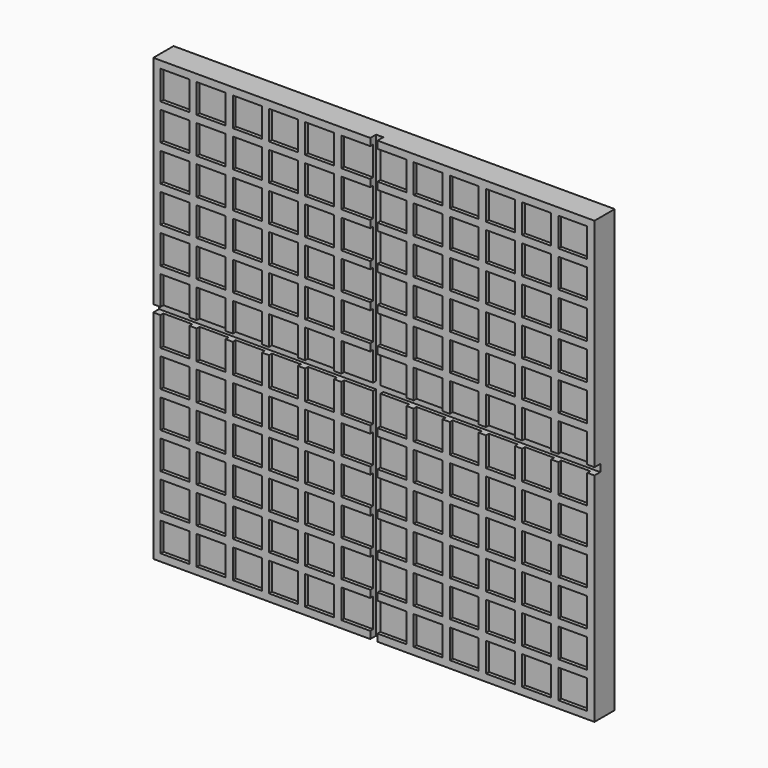
from build123d import *

# Parameters (mm, degrees)
F0_W     = 122
F0_H     = 122
F2_DEPTH = 7
F1_W     = 60
F1_H     = 2
F1_W_2   = 2
F1_H_2   = 60
F3_DEPTH = 7
F4_W     = 8
F4_H     = 8
F5_DEPTH = 1
F6_W     = 60
F6_H     = 2
F6_W_2   = 2
F6_H_2   = 60
F7_DEPTH = 2


# Not quite as in the source:
# - a feature names something its author has since deleted; it is built from what else it names


with BuildPart() as f2:
    # F0 (on Front) → F2 (new body)
    with BuildSketch(Plane.XZ):
        Rectangle(F0_W, F0_H)
    extrude(amount=F2_DEPTH)

    # F1 (on Front) → F3 (join, through all)
    with BuildSketch(Plane.XZ):
        with Locations((-31, 0)):
            Rectangle(F1_W, F1_H)
        with Locations((0, 31)):
            Rectangle(F1_W_2, F1_H_2)
        Rectangle(F1_W_2, F1_H)
        with Locations((31, 0)):
            Rectangle(F1_W, F1_H)
        with Locations((0, -31)):
            Rectangle(F1_W_2, F1_H_2)
    extrude(amount=F3_DEPTH)

    # F4 (on face) → F5 (cut)
    with BuildSketch(Plane.XZ.offset(7)):
        with Locations((-55, -55)):
            Rectangle(F4_W, F4_H)
        with Locations((-55, -45)):
            Rectangle(F4_W, F4_H)
        with Locations((-55, -35)):
            Rectangle(F4_W, F4_H)
        with Locations((-55, -25)):
            Rectangle(F4_W, F4_H)
        with Locations((-55, -15)):
            Rectangle(F4_W, F4_H)
        with Locations((-55, -5)):
            Rectangle(F4_W, F4_H)
        with Locations((-55, 5)):
            Rectangle(F4_W, F4_H)
        with Locations((-55, 15)):
            Rectangle(F4_W, F4_H)
        with Locations((-55, 25)):
            Rectangle(F4_W, F4_H)
        with Locations((-55, 35)):
            Rectangle(F4_W, F4_H)
        with Locations((-55, 45)):
            Rectangle(F4_W, F4_H)
        with Locations((-45, -55)):
            Rectangle(F4_W, F4_H)
        with Locations((-45, -45)):
            Rectangle(F4_W, F4_H)
        with Locations((-45, -35)):
            Rectangle(F4_W, F4_H)
        with Locations((-45, -25)):
            Rectangle(F4_W, F4_H)
        with Locations((-45, -15)):
            Rectangle(F4_W, F4_H)
        with Locations((-45, -5)):
            Rectangle(F4_W, F4_H)
        with Locations((-45, 5)):
            Rectangle(F4_W, F4_H)
        with Locations((-45, 15)):
            Rectangle(F4_W, F4_H)
        with Locations((-45, 25)):
            Rectangle(F4_W, F4_H)
        with Locations((-45, 35)):
            Rectangle(F4_W, F4_H)
        with Locations((-45, 45)):
            Rectangle(F4_W, F4_H)
        with Locations((-35, -55)):
            Rectangle(F4_W, F4_H)
        with Locations((-35, -45)):
            Rectangle(F4_W, F4_H)
        with Locations((-35, -35)):
            Rectangle(F4_W, F4_H)
        with Locations((-35, -25)):
            Rectangle(F4_W, F4_H)
        with Locations((-35, -15)):
            Rectangle(F4_W, F4_H)
        with Locations((-35, -5)):
            Rectangle(F4_W, F4_H)
        with Locations((-35, 5)):
            Rectangle(F4_W, F4_H)
        with Locations((-35, 15)):
            Rectangle(F4_W, F4_H)
        with Locations((-35, 25)):
            Rectangle(F4_W, F4_H)
        with Locations((-35, 35)):
            Rectangle(F4_W, F4_H)
        with Locations((-35, 45)):
            Rectangle(F4_W, F4_H)
        with Locations((-25, -55)):
            Rectangle(F4_W, F4_H)
        with Locations((-25, -45)):
            Rectangle(F4_W, F4_H)
        with Locations((-25, -35)):
            Rectangle(F4_W, F4_H)
        with Locations((-25, -25)):
            Rectangle(F4_W, F4_H)
        with Locations((-25, -15)):
            Rectangle(F4_W, F4_H)
        with Locations((-25, -5)):
            Rectangle(F4_W, F4_H)
        with Locations((-25, 5)):
            Rectangle(F4_W, F4_H)
        with Locations((-25, 15)):
            Rectangle(F4_W, F4_H)
        with Locations((-25, 25)):
            Rectangle(F4_W, F4_H)
        with Locations((-25, 35)):
            Rectangle(F4_W, F4_H)
        with Locations((-25, 45)):
            Rectangle(F4_W, F4_H)
        with Locations((-15, -55)):
            Rectangle(F4_W, F4_H)
        with Locations((-15, -45)):
            Rectangle(F4_W, F4_H)
        with Locations((-15, -35)):
            Rectangle(F4_W, F4_H)
        with Locations((-15, -25)):
            Rectangle(F4_W, F4_H)
        with Locations((-15, -15)):
            Rectangle(F4_W, F4_H)
        with Locations((-15, -5)):
            Rectangle(F4_W, F4_H)
        with Locations((-15, 5)):
            Rectangle(F4_W, F4_H)
        with Locations((-15, 15)):
            Rectangle(F4_W, F4_H)
        with Locations((-15, 25)):
            Rectangle(F4_W, F4_H)
        with Locations((-15, 35)):
            Rectangle(F4_W, F4_H)
        with Locations((-15, 45)):
            Rectangle(F4_W, F4_H)
        with Locations((-5, -55)):
            Rectangle(F4_W, F4_H)
        with Locations((-5, -45)):
            Rectangle(F4_W, F4_H)
        with Locations((-5, -35)):
            Rectangle(F4_W, F4_H)
        with Locations((-5, -25)):
            Rectangle(F4_W, F4_H)
        with Locations((-5, -15)):
            Rectangle(F4_W, F4_H)
        with Locations((-5, -5)):
            Rectangle(F4_W, F4_H)
        with Locations((-5, 5)):
            Rectangle(F4_W, F4_H)
        with Locations((-5, 15)):
            Rectangle(F4_W, F4_H)
        with Locations((-5, 25)):
            Rectangle(F4_W, F4_H)
        with Locations((-5, 35)):
            Rectangle(F4_W, F4_H)
        with Locations((-5, 45)):
            Rectangle(F4_W, F4_H)
        with Locations((5, -55)):
            Rectangle(F4_W, F4_H)
        with Locations((5, -45)):
            Rectangle(F4_W, F4_H)
        with Locations((5, -35)):
            Rectangle(F4_W, F4_H)
        with Locations((5, -25)):
            Rectangle(F4_W, F4_H)
        with Locations((5, -15)):
            Rectangle(F4_W, F4_H)
        with Locations((5, -5)):
            Rectangle(F4_W, F4_H)
        with Locations((5, 5)):
            Rectangle(F4_W, F4_H)
        with Locations((5, 15)):
            Rectangle(F4_W, F4_H)
        with Locations((5, 25)):
            Rectangle(F4_W, F4_H)
        with Locations((5, 35)):
            Rectangle(F4_W, F4_H)
        with Locations((5, 45)):
            Rectangle(F4_W, F4_H)
        with Locations((15, -55)):
            Rectangle(F4_W, F4_H)
        with Locations((15, -45)):
            Rectangle(F4_W, F4_H)
        with Locations((15, -35)):
            Rectangle(F4_W, F4_H)
        with Locations((15, -25)):
            Rectangle(F4_W, F4_H)
        with Locations((15, -15)):
            Rectangle(F4_W, F4_H)
        with Locations((15, -5)):
            Rectangle(F4_W, F4_H)
        with Locations((15, 5)):
            Rectangle(F4_W, F4_H)
        with Locations((15, 15)):
            Rectangle(F4_W, F4_H)
        with Locations((15, 25)):
            Rectangle(F4_W, F4_H)
        with Locations((15, 35)):
            Rectangle(F4_W, F4_H)
        with Locations((15, 45)):
            Rectangle(F4_W, F4_H)
        with Locations((25, -55)):
            Rectangle(F4_W, F4_H)
        with Locations((25, -45)):
            Rectangle(F4_W, F4_H)
        with Locations((25, -35)):
            Rectangle(F4_W, F4_H)
        with Locations((25, -25)):
            Rectangle(F4_W, F4_H)
        with Locations((25, -15)):
            Rectangle(F4_W, F4_H)
        with Locations((25, -5)):
            Rectangle(F4_W, F4_H)
        with Locations((25, 5)):
            Rectangle(F4_W, F4_H)
        with Locations((25, 15)):
            Rectangle(F4_W, F4_H)
        with Locations((25, 25)):
            Rectangle(F4_W, F4_H)
        with Locations((25, 35)):
            Rectangle(F4_W, F4_H)
        with Locations((25, 45)):
            Rectangle(F4_W, F4_H)
        with Locations((35, -55)):
            Rectangle(F4_W, F4_H)
        with Locations((35, -45)):
            Rectangle(F4_W, F4_H)
        with Locations((35, -35)):
            Rectangle(F4_W, F4_H)
        with Locations((35, -25)):
            Rectangle(F4_W, F4_H)
        with Locations((35, -15)):
            Rectangle(F4_W, F4_H)
        with Locations((35, -5)):
            Rectangle(F4_W, F4_H)
        with Locations((35, 5)):
            Rectangle(F4_W, F4_H)
        with Locations((35, 15)):
            Rectangle(F4_W, F4_H)
        with Locations((35, 25)):
            Rectangle(F4_W, F4_H)
        with Locations((35, 35)):
            Rectangle(F4_W, F4_H)
        with Locations((35, 45)):
            Rectangle(F4_W, F4_H)
        with Locations((45, -55)):
            Rectangle(F4_W, F4_H)
        with Locations((45, -45)):
            Rectangle(F4_W, F4_H)
        with Locations((45, -35)):
            Rectangle(F4_W, F4_H)
        with Locations((45, -25)):
            Rectangle(F4_W, F4_H)
        with Locations((45, -15)):
            Rectangle(F4_W, F4_H)
        with Locations((45, -5)):
            Rectangle(F4_W, F4_H)
        with Locations((45, 5)):
            Rectangle(F4_W, F4_H)
        with Locations((45, 15)):
            Rectangle(F4_W, F4_H)
        with Locations((45, 25)):
            Rectangle(F4_W, F4_H)
        with Locations((45, 35)):
            Rectangle(F4_W, F4_H)
        with Locations((45, 45)):
            Rectangle(F4_W, F4_H)
        with Locations((55, -55)):
            Rectangle(F4_W, F4_H)
        with Locations((55, -45)):
            Rectangle(F4_W, F4_H)
        with Locations((55, -35)):
            Rectangle(F4_W, F4_H)
        with Locations((55, -25)):
            Rectangle(F4_W, F4_H)
        with Locations((55, -15)):
            Rectangle(F4_W, F4_H)
        with Locations((55, -5)):
            Rectangle(F4_W, F4_H)
        with Locations((55, 5)):
            Rectangle(F4_W, F4_H)
        with Locations((55, 15)):
            Rectangle(F4_W, F4_H)
        with Locations((55, 25)):
            Rectangle(F4_W, F4_H)
        with Locations((55, 35)):
            Rectangle(F4_W, F4_H)
        with Locations((55, 45)):
            Rectangle(F4_W, F4_H)
        with Locations((-55, 55)):
            Rectangle(F4_W, F4_H)
        with Locations((-45, 55)):
            Rectangle(F4_W, F4_H)
        with Locations((-35, 55)):
            Rectangle(F4_W, F4_H)
        with Locations((-25, 55)):
            Rectangle(F4_W, F4_H)
        with Locations((-15, 55)):
            Rectangle(F4_W, F4_H)
        with Locations((-5, 55)):
            Rectangle(F4_W, F4_H)
        with Locations((5, 55)):
            Rectangle(F4_W, F4_H)
        with Locations((15, 55)):
            Rectangle(F4_W, F4_H)
        with Locations((25, 55)):
            Rectangle(F4_W, F4_H)
        with Locations((35, 55)):
            Rectangle(F4_W, F4_H)
        with Locations((45, 55)):
            Rectangle(F4_W, F4_H)
        with Locations((55, 55)):
            Rectangle(F4_W, F4_H)
    extrude(amount=-F5_DEPTH, mode=Mode.SUBTRACT)

    # F6 (on face) → F7 (cut)
    with BuildSketch(Plane.XZ.offset(7)):
        with Locations((-31, 0)):
            Rectangle(F6_W, F6_H)
        with Locations((0, 31)):
            Rectangle(F6_W_2, F6_H_2)
        Rectangle(F6_W_2, F6_H)
        with Locations((31, 0)):
            Rectangle(F6_W, F6_H)
        with Locations((0, -31)):
            Rectangle(F6_W_2, F6_H_2)
    extrude(amount=-F7_DEPTH, mode=Mode.SUBTRACT)


solid = f2.part
